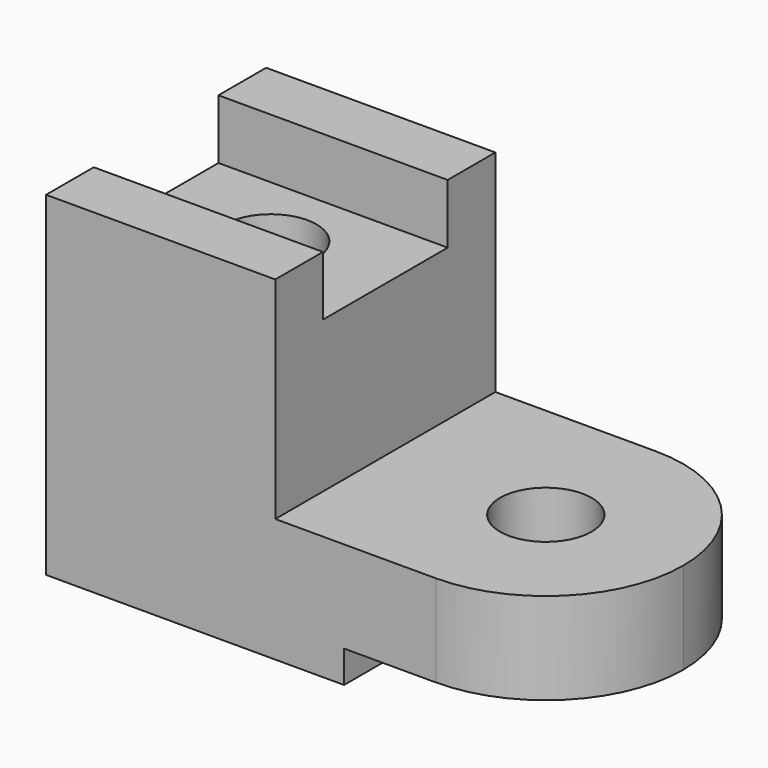
from build123d import *

# Parameters (mm, degrees)
F1_DEPTH  = 60
F2_W      = 50
F2_H      = 13
F3_DEPTH  = 13
F4_W      = 50
F4_H      = 13
F5_DEPTH  = 13
F6_R      = 29.99999
F7_R      = 10
F9_DEPTH  = 20
F8_R      = 10
F10_DEPTH = 60


# Not quite as in the source:
# - a fillet or chamfer is up to 0.001 mm smaller than in the source, because OpenCascade refuses the exact size


with BuildPart() as f1:
    # F0 (on Front) → F1 (new body)
    with BuildSketch(Plane.XZ):
        Polygon((-44.2382382879, 60), (-44.2382382879, 0), (20.7617617121, 0), (20.7617617121, 7), (70.7617617121, 7), (70.7617617121, 27), (5.7617617121, 27), (5.7617617121, 60), align=None)
    extrude(amount=F1_DEPTH)

    # F2 (on face) → F3 (join)
    with BuildSketch(Plane.XY.offset(60)):
        with Locations((-19.2382382879, -6.5)):
            Rectangle(F2_W, F2_H)
    extrude(amount=F3_DEPTH)

    # F4 (on face) → F5 (join)
    with BuildSketch(Plane.XY.offset(60)):
        with Locations((-19.2382382879, -53.5)):
            Rectangle(F4_W, F4_H)
    extrude(amount=F5_DEPTH)

    # F6 (radius 30 in the source; OpenCascade refuses exactly that, so slightly less here)
    f6_edges = [f1.edges().sort_by_distance(p)[0] for p in [
        (70.761762, -60, 17),
        (70.761762, 0, 17),
    ]]
    fillet(f6_edges, radius=F6_R)

    # F7 (on face) → F9 (cut)
    with BuildSketch(Plane.XY.offset(27)):
        with Locations((40.7617617121, -30)):
            Circle(F7_R)
    extrude(amount=-F9_DEPTH, mode=Mode.SUBTRACT)

    # F8 (on face) → F10 (cut)
    with BuildSketch(Plane.XY.offset(60)):
        with Locations((-19.2382382879, -30)):
            Circle(F8_R)
    extrude(amount=-F10_DEPTH, mode=Mode.SUBTRACT)


solid = f1.part
